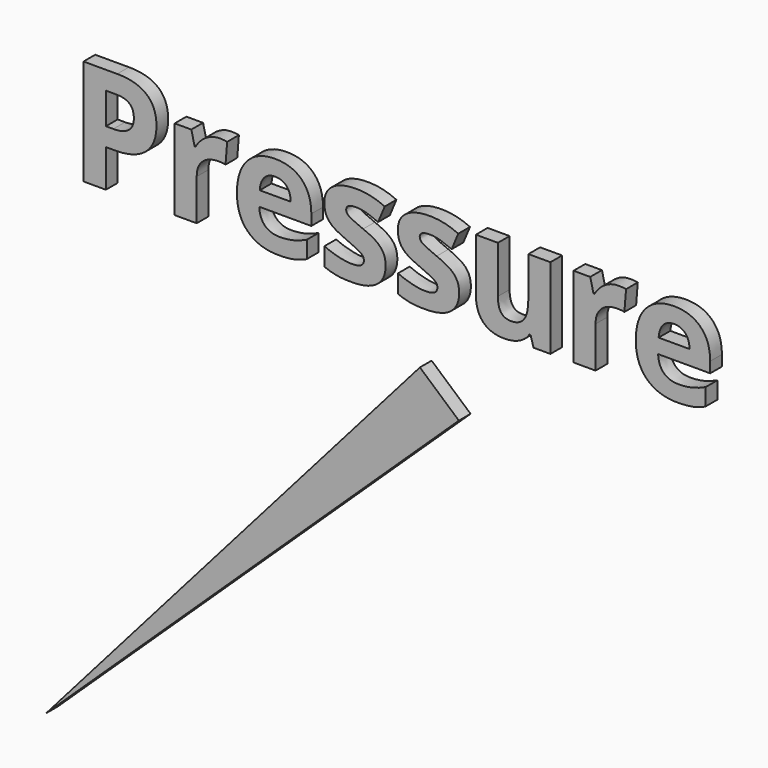
from build123d import *

# Parameters (mm, degrees)
F0_TEXT_SIZE = 12.826845826
F1_DEPTH     = 1.27


# Not quite as in the source:
# - Text() gives the source's letters only with a copy of the font that has no kerning and outlines rounded to 1/6400 em; it was checked with that copy


with BuildPart() as f1:
    # F0 (on Front) → F1 (new body)
    with BuildSketch(Plane.XZ):
        Polygon((2.1264876705, 5.2546160296), (-30.2842967212, -31.6867046058), (5.5038728978, 2.2914381429), align=None)
        with Locations((-28.1932794314, 9.9594080821)):
            Text('Pressure', F0_TEXT_SIZE, font='Open Sans', font_style=FontStyle.BOLD, text_align=(TextAlign.LEFT, TextAlign.BOTTOM))
    extrude(amount=F1_DEPTH)


solid = f1.part
